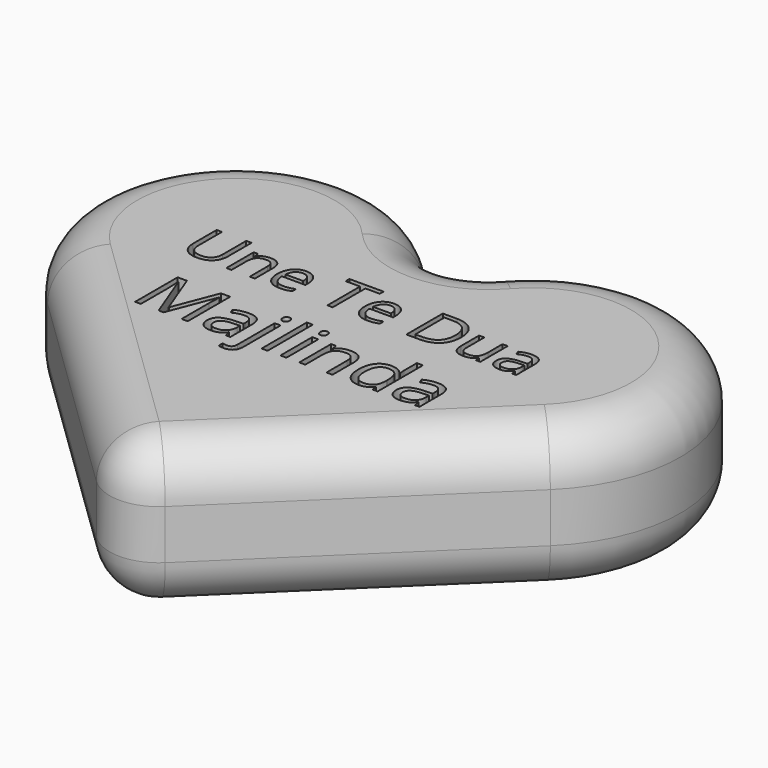
from build123d import *

# Parameters (mm, degrees)
F1_DEPTH       = 19.05
F2_TEXT_SIZE   = 16.4031597763
F2_TEXT_SIZE_2 = 19.1247058824
F3_DEPTH       = 38.101
F4_R           = 12.7


# Not quite as in the source:
# - Text() gives the source's letters only with a copy of the font that has no kerning and outlines rounded to 1/6400 em; it was checked with that copy


with BuildPart() as f1:
    # F0 (on Top) → F1 (new body, symmetric)
    with BuildSketch(Plane.XY):
        with BuildLine():
            ThreePointArc((64.6135011408, 10.7386356835), (52.956742687, 73.1840020056), (0, 38.1))
            ThreePointArc((0, 38.1), (-52.956742687, 73.1840020056), (-64.6135011408, 10.7386356835))
            Line((-64.6135011408, 10.7386356835), (0, -51.8726477448))
            Line((0, -51.8726477448), (64.6135011408, 10.7386356835))
        make_face()
    extrude(amount=F1_DEPTH, both=True)

    # F2 (on face) → F3 (cut, through all)
    with BuildSketch(Plane.XY.offset(19.05)):
        with Locations((-44.45, 26.2897249611)):
            Text('Une Te Dua', F2_TEXT_SIZE, font='Open Sans', text_align=(TextAlign.LEFT, TextAlign.BOTTOM))
        with Locations((-38.1, 3.3752117647)):
            Text('Majlinda', F2_TEXT_SIZE_2, font='Open Sans', text_align=(TextAlign.LEFT, TextAlign.BOTTOM))
    extrude(amount=-F3_DEPTH, mode=Mode.SUBTRACT)

    # F4
    f4_edges = [f1.edges().sort_by_distance(p)[0] for p in [
        (0, 38.1, 0),
        (-52.956743, 73.184002, -19.05),
        (-64.613501, 10.738636, 0),
        (-52.956743, 73.184002, 19.05),
        (-32.306751, -20.567006, -19.05),
        (0, -51.872648, 0),
        (-32.306751, -20.567006, 19.05),
        (52.956743, 73.184002, -19.05),
        (52.956743, 73.184002, 19.05),
        (64.613501, 10.738636, 0),
        (32.306751, -20.567006, -19.05),
        (32.306751, -20.567006, 19.05),
    ]]
    fillet(f4_edges, radius=F4_R)


solid = f1.part
